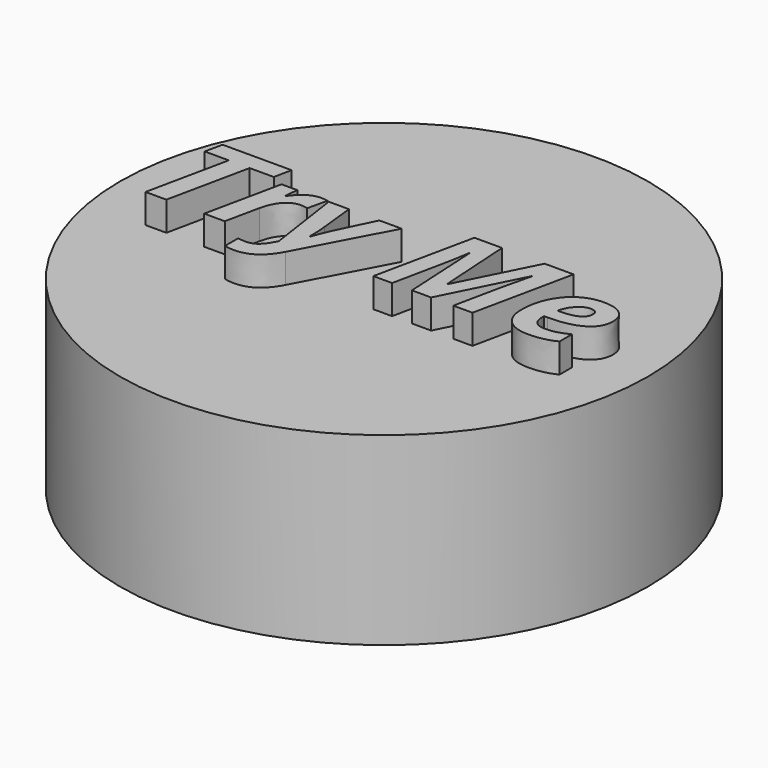
from build123d import *

# Parameters (mm, degrees)
F0_R         = 20
F1_DEPTH     = 14
F2_TEXT_SIZE = 10.6034606391
F3_DEPTH     = 2.2098


# Not quite as in the source:
# - Text() gives the source's letters only with a copy of the font that has no kerning and outlines rounded to 1/6400 em; it was checked with that copy


with BuildPart() as f1:
    # F0 (on Top) → F1 (new body)
    with BuildSketch(Plane.XY):
        Circle(F0_R)
    extrude(amount=F1_DEPTH)

    # F2 (on face) → F3 (join)
    with BuildSketch(Plane.XY.offset(14)):
        with Locations((-16.6995050601, -3.4188913024)):
            Text('Try Me', F2_TEXT_SIZE, font='Open Sans', font_style=FontStyle.BOLDITALIC, text_align=(TextAlign.LEFT, TextAlign.BOTTOM))
    extrude(amount=F3_DEPTH)


solid = f1.part
